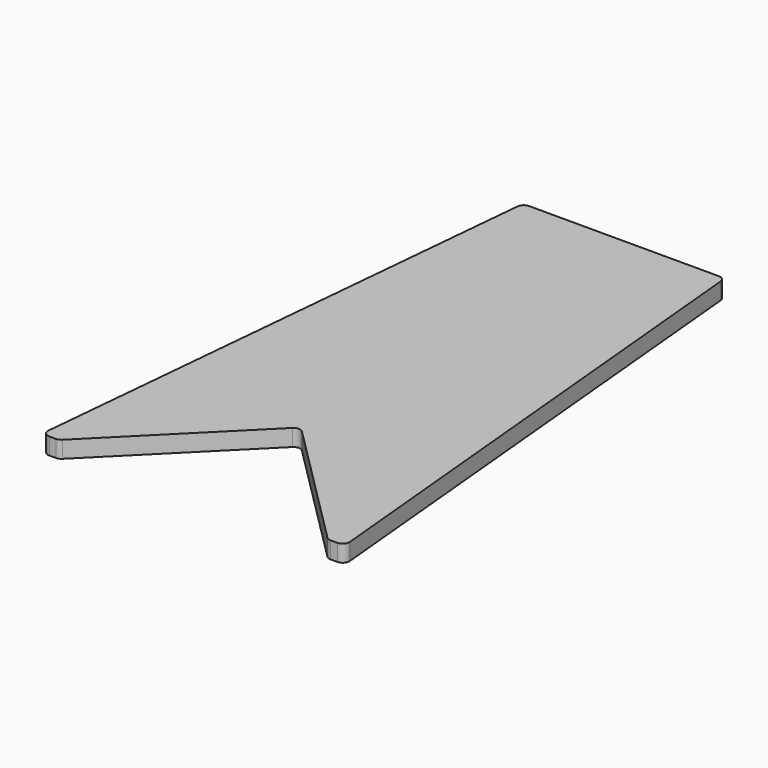
from build123d import *

# Parameters (mm, degrees)
F1_DEPTH = 6.35
F3_DEPTH = 6.351
F4_R     = 2.54


with BuildPart() as f1:
    # F0 (on Top) → F1 (new body)
    with BuildSketch(Plane.XY):
        Polygon((-38.1, 203.2), (-57.15, 0), (57.15, 0), (38.1, 203.2), align=None)
    extrude(amount=F1_DEPTH)

    # F2 (on face) → F3 (cut, through all)
    with BuildSketch(Plane.XY.offset(6.35)):
        Polygon((0, 50.8), (-50.8, 0), (50.8, 0), align=None)
    extrude(amount=-F3_DEPTH, mode=Mode.SUBTRACT)

    # F4
    f4_edges = [f1.edges().sort_by_distance(p)[0] for p in [
        (-38.1, 203.2, 3.175),
        (38.1, 203.2, 3.175),
        (0, 50.8, 3.175),
        (-50.8, 0, 3.175),
        (-57.15, 0, 3.175),
        (50.8, 0, 3.175),
        (57.15, 0, 3.175),
    ]]
    fillet(f4_edges, radius=F4_R)


solid = f1.part
